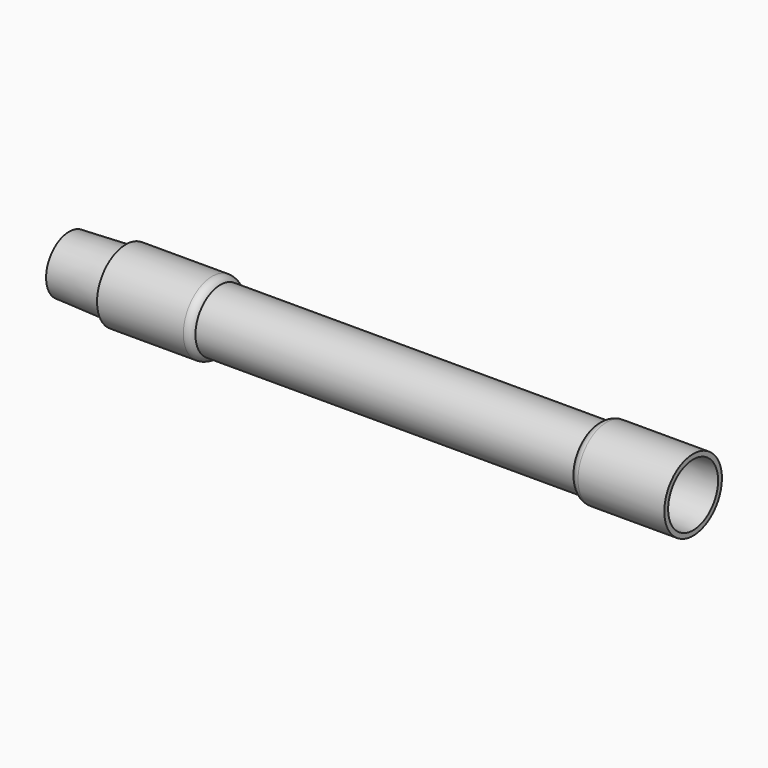
from build123d import *


# Not quite as in the source:
# - a fillet or chamfer that OpenCascade refuses, or shapes differently, is made with other operations: its cross-section is extruded or revolved along the edge and cut away or added


with BuildPart() as f2:
    # F0 (on Front) → F2 (revolve)
    with BuildSketch(Plane.XZ):
        Polygon((0, 15.24), (0, 12.7), (30, 12.7), (290, 12.7), (290, 13.97), (330, 16.51), (330, 19.05), (280, 19.05), (280, 16.51), (80, 16.51), (80, 19.05), (30, 19.05), (30, 16.51), align=None)
    revolve(axis=Axis((0, 0, 0), (1, 0, 0)))

    # F3: fillet of radius 5 on 2 edges, made by hand

    # F3_s1 → F3_t2 (revolve, cut)
    with BuildSketch(Plane.XZ):
        with BuildLine():
            ThreePointArc((80, 16.51), (78.1669446402, 18.3685645763), (75.6470240065, 19.05))
            Line((75.6470240065, 19.05), (75.6470240065, 19.15))
            Line((75.6470240065, 19.15), (80, 19.15))
            Line((80, 19.15), (80.1, 19.05))
            ThreePointArc((80.1, 19.05), (80.1, 17.78), (80.0870595199, 16.5592))
            Line((80.0870595199, 16.5592), (80, 16.51))
        make_face()
    revolve(axis=Axis((80, 0, 0), (1, 0, 0)), mode=Mode.SUBTRACT)

    # F3_s3 → F3_t4 (revolve, cut)
    with BuildSketch(Plane.XZ):
        with BuildLine():
            ThreePointArc((284.3529759935, 19.05), (281.8330553598, 18.3685645763), (280, 16.51))
            Line((280, 16.51), (279.9129404801, 16.5592))
            ThreePointArc((279.9129404801, 16.5592), (279.9, 17.78), (279.9, 19.05))
            Line((279.9, 19.05), (280, 19.15))
            Line((280, 19.15), (284.3529759935, 19.15))
            Line((284.3529759935, 19.15), (284.3529759935, 19.05))
        make_face()
    revolve(axis=Axis((280, 0, 0), (1, 0, 0)), mode=Mode.SUBTRACT)


solid = f2.part
